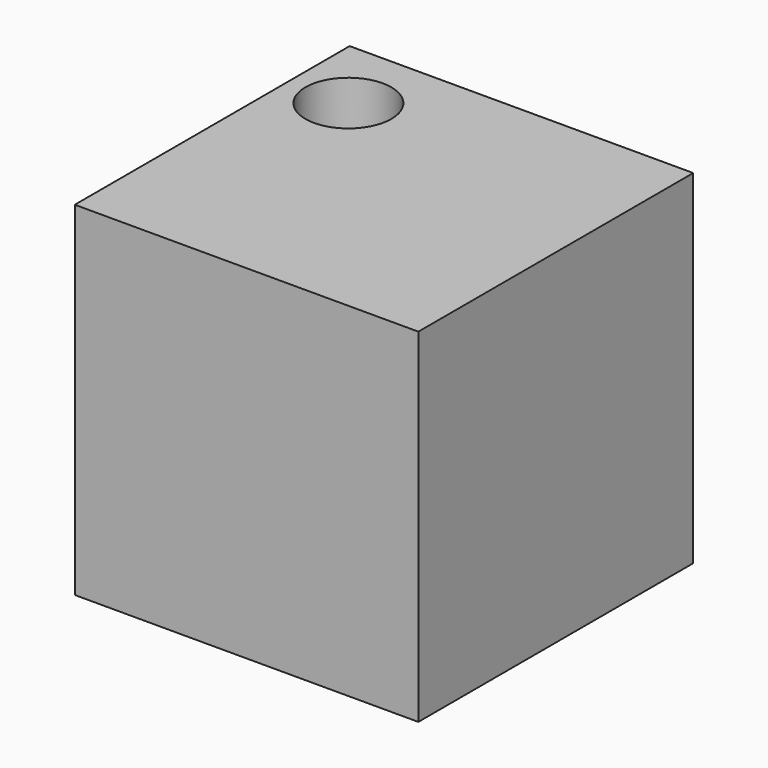
from build123d import *

# Parameters (mm, degrees)
F1_W     = 101.6
F1_H     = 101.6
F2_DEPTH = 50.8
F3_R     = 12.7
F4_DEPTH = 25.4
F5_R     = 12.7
F6_DEPTH = 17.78


# Not quite as in the source:
# - a variable given as a bare number and used for a length is read in inches; the dataset says mm whatever the document's units were


with BuildPart() as f2:
    # F1 (on Front) → F2 (new body, symmetric)
    with BuildSketch(Plane.XZ):
        Rectangle(F1_W, F1_H)
    extrude(amount=F2_DEPTH, both=True)

    # F3 (on face) → F4 (cut)
    with BuildSketch(Plane.XY.offset(50.8)):
        with Locations((-33.2122892141, 28.3519532531)):
            Circle(F3_R)
    extrude(amount=-F4_DEPTH, mode=Mode.SUBTRACT)

    # F5 (on face) → F6 (join)
    with BuildSketch(Plane(origin=(0, 0, -50.8), x_dir=(1, 0, 0), z_dir=(0, 0, -1))):
        with Locations((-33.2122892141, -28.3519532531)):
            Circle(F5_R)
    extrude(amount=F6_DEPTH)


solid = f2.part
